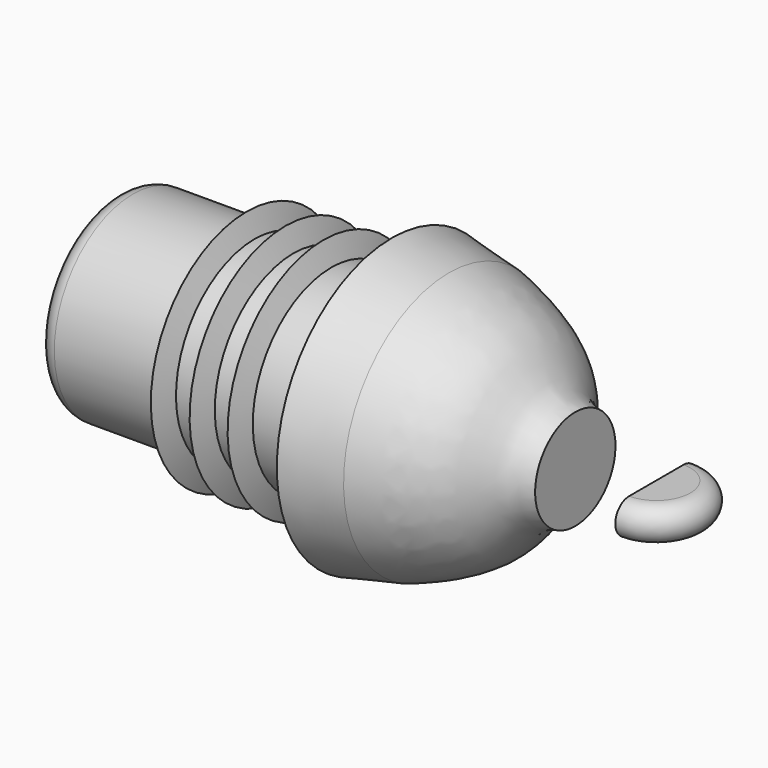
from build123d import *

# Parameters (mm, degrees)
F3_ANGLE_BACK = 90
F3_ANGLE      = 180
F5_R          = 1.5


# Not quite as in the source:
# - the program builds the solid bodies; features that only make, move or delete a surface that nothing else refers to are left out


with BuildPart() as f1:
    # F0 (on Front) → F1 (revolve)
    with BuildSketch(Plane.XZ):
        Polygon((-6.5773623064, 8.5310461), (-5.2633433491, 8.5310461), (-5.9452718124, 10.4112434772), align=None)
        with BuildLine():
            Line((0, 12.5), (-2.086e-07, 8.5310461))
            Line((-2.086e-07, 8.5310461), (-5.2633433491, 8.5310461))
            Line((-5.2633433491, 8.5310461), (-6.5773623064, 8.5310461))
            Line((-6.5773623064, 8.5310461), (-8.5633396059, 8.5310461))
            Line((-8.5633396059, 8.5310461), (-9.8773585632, 8.5310461))
            Line((-9.8773585632, 8.5310461), (-11.9312460423, 8.5310461))
            Line((-11.9312460423, 8.5310461), (-13.2452649996, 8.5310461))
            Line((-13.2452649996, 8.5310461), (-24.0000002086, 8.5310461))
            Line((-24.0000002086, 8.5310461), (-24.0000002086, 6.969221402))
            Line((-24.0000002086, 6.969221402), (4.2684120126, 6.969221402))
            Line((4.2684120126, 6.969221402), (14.3519612029, 3.2055957709))
            Line((14.3519612029, 3.2055957709), (14.3519612029, 0))
            Line((14.3519612029, 0), (15.9248222774, 0))
            Line((15.9248222774, 0), (15.9248222774, 4.3634505053))
            add(Edge.make_bspline(
                [(4.947933834, 11.4384293556), (5.9793661215, 11.0697915829), (8.0593561798, 10.3198783934), (11.2462916486, 8.5163300937), (12.8397611568, 6.2322058814), (13.8845362692, 5.0202002888), (15.0923938592, 4.5281993111), (15.8833928624, 4.2969274606), (15.9231948476, 4.3586775517), (15.9248222774, 4.3634505053)],
                knots=[0, 0, 0, 0, 0.204407807, 0.4182345345, 0.6036515616, 0.742726845, 0.8743332982, 0.9688664238, 0.9757506271, 0.9757506271, 0.9757506271, 0.9757506271], degree=3))
            Line((4.947933834, 11.4384293556), (0, 12.5))
        make_face()
        Polygon((-9.8773585632, 8.5310461), (-8.5633396059, 8.5310461), (-9.2452680692, 10.4112434772), align=None)
        Polygon((-13.2452649996, 8.5310461), (-11.9312460423, 8.5310461), (-12.6131745055, 10.4112434772), align=None)
    revolve(axis=Axis((-3.8916748017, 0, 0), (1, 0, 0)))

    # F5
    f5_edges = [f1.edges().sort_by_distance(p)[0] for p in [
        (-24, 0, -8.531046),
    ]]
    fillet(f5_edges, radius=F5_R)


with BuildPart() as f3:
    # F2 (on Front) → F3 (revolve)
    with BuildSketch(Plane.XZ, mode=Mode.PRIVATE) as f3_sk:
        with BuildLine():
            Line((22.9624137282, 1.4185722424), (22.9624137282, -1.5814277576))
            Line((22.9624137282, -1.5814277576), (25.9165772951, -1.5814277576))
            ThreePointArc((25.9165772951, -1.5814277576), (27.4165772951, -0.0814277576), (25.9165772951, 1.4185722424))
            Line((25.9165772951, 1.4185722424), (22.9624137282, 1.4185722424))
        make_face()
    revolve(f3_sk.sketch.rotate(Axis((22.9624137282, 0, -0.0814277576), (0, 0, 1)), -F3_ANGLE_BACK), axis=Axis((22.9624137282, 0, -0.0814277576), (0, 0, 1)), revolution_arc=F3_ANGLE)


solid = Compound([f1.part, f3.part])
